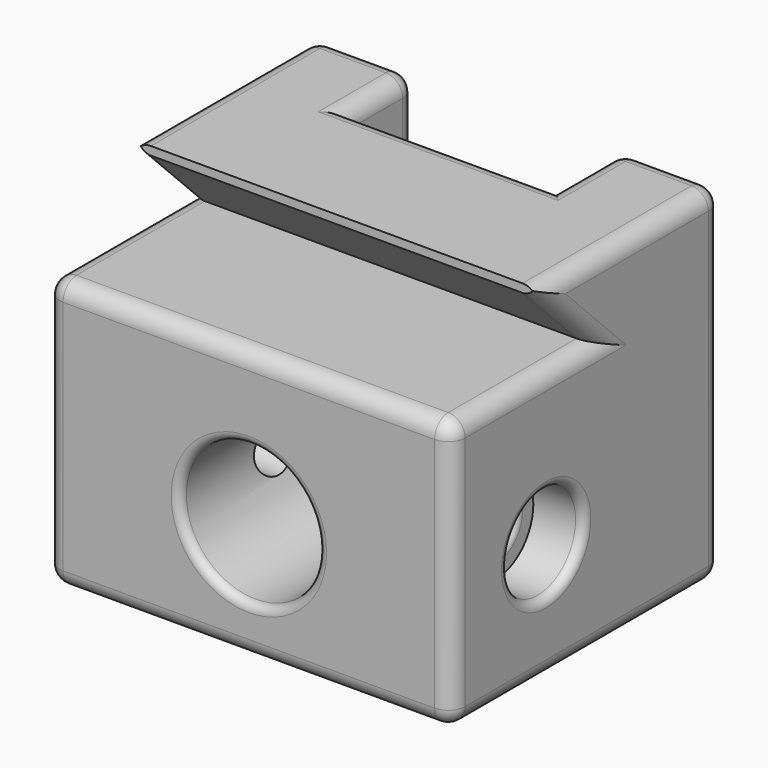
from build123d import *

# Parameters (mm, degrees)
F0_W           = 24
F0_H           = 20
F1_DEPTH       = 18.5
F2_R           = 1.5
F3_DEPTH       = 25
F4_DEPTH       = 2
F5_R           = 4.1
F6_DEPTH       = 25
F7_W           = 12.2
F7_H           = 5
F8_DEPTH       = 25
F9_R           = 2.8
F9_R_2         = 1.5
F10_DEPTH      = 3
F12_DEPTH      = 10.5
F13_T1_DEPTH   = 22
F13_T3_DEPTH   = 15
F13_T5_DEPTH   = 18.5
F13_T7_DEPTH   = 3.9
F13_T9_DEPTH   = 14
F13_T11_DEPTH  = 3.9
F13_T13_DEPTH  = 4
F13_T15_DEPTH  = 12.2
F13_T17_DEPTH  = 18
F13_T19_DEPTH  = 2.75
F13_T21_DEPTH  = 5.5
F13_S25_W      = 1
F13_S25_H      = 1
F13_T26_DEPTH  = 1
F13_S31_W      = 1
F13_S31_H      = 1
F13_T32_DEPTH  = 1
F13_S37_W      = 1
F13_S37_H      = 1
F13_T38_DEPTH  = 1
F13_S43_W      = 1
F13_S43_H      = 1
F13_T44_DEPTH  = 1
F13_S49_W      = 1
F13_S49_H      = 1
F13_T50_DEPTH  = 1
F13_S55_W      = 1
F13_S55_H      = 1
F13_T56_DEPTH  = 1
F13_S61_W      = 1
F13_S61_H      = 1
F13_T62_DEPTH  = 1
F13_S67_W      = 1
F13_S67_H      = 1
F13_T68_DEPTH  = 1
F13_S73_W      = 1
F13_S73_H      = 1
F13_T74_DEPTH  = 1
F13_S79_W      = 1
F13_S79_H      = 1
F13_T80_DEPTH  = 1
F13_S85_W      = 1
F13_S85_H      = 1
F13_T86_DEPTH  = 1
F13_S91_W      = 1
F13_S91_H      = 1
F13_T92_DEPTH  = 1
F13_T98_DEPTH  = 12
F13_T103_DEPTH = 12
F13_T108_DEPTH = 10.6568542495
F13_T113_DEPTH = 10.6568542495
F13_T119_DEPTH = 12
F13_T123_DEPTH = 10.6568542495
F13_T130_DEPTH = 12
F13_T134_DEPTH = 10.6568542495
F13_T141_DEPTH = 6.5
F13_T145_DEPTH = 14.7
F13_T152_DEPTH = 14.7
F13_T156_DEPTH = 6.5
F13_T163_DEPTH = 6.5
F13_T167_DEPTH = 14.7
F13_T174_DEPTH = 6.5
F13_T178_DEPTH = 14.7
F13_T185_DEPTH = 5.25
F13_T189_DEPTH = 8
F13_T196_DEPTH = 8
F13_T200_DEPTH = 5.25
F13_T207_DEPTH = 8
F13_T211_DEPTH = 5.25
F13_T218_DEPTH = 8
F13_T222_DEPTH = 5.25
F14_R          = 0.5


# Not quite as in the source:
# - a fillet or chamfer that OpenCascade refuses, or shapes differently, is made with other operations: its cross-section is extruded or revolved along the edge and cut away or added


with BuildPart() as f1:
    # F0 (on Top) → F1 (new body)
    with BuildSketch(Plane.XY):
        Rectangle(F0_W, F0_H)
    extrude(amount=F1_DEPTH)

    # F2 (on face) → F3 (cut)
    with BuildSketch(Plane(origin=(-12, 0, 0), x_dir=(0, -1, 0), z_dir=(-1, 0, 0))):
        Polygon((-0.5, 14), (10, 14), (10, 18.5), (3.5, 18.5), (3.5, 18), align=None)
        with Locations((3, 5)):
            Circle(F2_R)
    extrude(amount=-F3_DEPTH, mode=Mode.SUBTRACT)

    # F4 (add): a face of the model
    f4_faces = [f1.faces().sort_by_distance(p)[0] for p in [
        (0, 0, 0),
    ]]
    extrude(f4_faces, amount=F4_DEPTH)

    # F5 (on face) → F6 (cut)
    with BuildSketch(Plane.XZ.offset(10)):
        with Locations((0, 5)):
            Circle(F5_R)
    extrude(amount=-F6_DEPTH, mode=Mode.SUBTRACT)

    # F7 (on face) → F8 (cut)
    with BuildSketch(Plane.XY.offset(18.5)):
        with Locations((0, 7.5)):
            Rectangle(F7_W, F7_H)
    extrude(amount=-F8_DEPTH, mode=Mode.SUBTRACT)

    # F9 (on face) → F10 (cut)
    with BuildSketch(Plane.YZ.offset(12)):
        with Locations((-3, 5)):
            Circle(F9_R)
        with Locations((-3, 5)):
            Circle(F9_R_2, mode=Mode.SUBTRACT)
    extrude(amount=-F10_DEPTH, mode=Mode.SUBTRACT)

    # F11 (on face) → F12 (cut)
    with BuildSketch(Plane(origin=(0, 0, -2), x_dir=(1, 0, 0), z_dir=(0, 0, -1))):
        Polygon((-7.05, 0.25), (-7.05, 3), (-7.05, 5.75), (-9.8, 5.75), (-9.8, 0.25), align=None)
    extrude(amount=-F12_DEPTH, mode=Mode.SUBTRACT)

    # F13: fillet of radius 1 on 30 edges, made by hand

    # F13_s2 → F13_t1 (cut)
    with BuildSketch(Plane.YZ.offset(-11)):
        with BuildLine():
            ThreePointArc((-10, 13), (-9.7071067812, 13.7071067812), (-9, 14))
            Line((-9, 14), (-10, 14))
            Line((-10, 14), (-10, 13))
        make_face()
        with BuildLine():
            ThreePointArc((-9, -2), (-9.7071067812, -1.7071067812), (-10, -1))
            Line((-10, -1), (-10, -2))
            Line((-10, -2), (-9, -2))
        make_face()
    extrude(amount=F13_T1_DEPTH, mode=Mode.SUBTRACT)

    # F13_s4 → F13_t3 (cut)
    with BuildSketch(Plane.XZ.offset(-9)):
        with BuildLine():
            ThreePointArc((-11, 18.5), (-11.7071067812, 18.2071067812), (-12, 17.5))
            Line((-12, 17.5), (-12, 18.5))
            Line((-12, 18.5), (-11, 18.5))
        make_face()
        with BuildLine():
            ThreePointArc((12, 17.5), (11.7071067812, 18.2071067812), (11, 18.5))
            Line((11, 18.5), (12, 18.5))
            Line((12, 18.5), (12, 17.5))
        make_face()
    extrude(amount=F13_T3_DEPTH, mode=Mode.SUBTRACT)

    # F13_s6 → F13_t5 (cut)
    with BuildSketch(Plane.XY.offset(-1)):
        with BuildLine():
            ThreePointArc((12, 9), (11.7071067812, 9.7071067812), (11, 10))
            Line((11, 10), (12, 10))
            Line((12, 10), (12, 9))
        make_face()
        with BuildLine():
            ThreePointArc((7.1, 10), (6.3928932188, 9.7071067812), (6.1, 9))
            Line((6.1, 9), (6.1, 10))
            Line((6.1, 10), (7.1, 10))
        make_face()
        with BuildLine():
            ThreePointArc((-7.1, 10), (-6.3928932188, 9.7071067812), (-6.1, 9))
            Line((-6.1, 9), (-6.1, 10))
            Line((-6.1, 10), (-7.1, 10))
        make_face()
        with BuildLine():
            ThreePointArc((-12, 9), (-11.7071067812, 9.7071067812), (-11, 10))
            Line((-11, 10), (-12, 10))
            Line((-12, 10), (-12, 9))
        make_face()
    extrude(amount=F13_T5_DEPTH, mode=Mode.SUBTRACT)

    # F13_s8 → F13_t7 (cut)
    with BuildSketch(Plane.YZ.offset(7.1)):
        with BuildLine():
            ThreePointArc((10, 17.5), (9.7071067812, 18.2071067812), (9, 18.5))
            Line((9, 18.5), (10, 18.5))
            Line((10, 18.5), (10, 17.5))
        make_face()
        with BuildLine():
            ThreePointArc((10, -1), (9.7071067812, -1.7071067812), (9, -2))
            Line((9, -2), (10, -2))
            Line((10, -2), (10, -1))
        make_face()
    extrude(amount=F13_T7_DEPTH, mode=Mode.SUBTRACT)

    # F13_s10 → F13_t9 (cut)
    with BuildSketch(Plane.XY.offset(-1)):
        with BuildLine():
            ThreePointArc((-11, -10), (-11.7071067812, -9.7071067812), (-12, -9))
            Line((-12, -9), (-12, -10))
            Line((-12, -10), (-11, -10))
        make_face()
        with BuildLine():
            ThreePointArc((12, -9), (11.7071067812, -9.7071067812), (11, -10))
            Line((11, -10), (12, -10))
            Line((12, -10), (12, -9))
        make_face()
    extrude(amount=F13_T9_DEPTH, mode=Mode.SUBTRACT)

    # F13_s12 → F13_t11 (cut)
    with BuildSketch(Plane.YZ.offset(-11)):
        with BuildLine():
            ThreePointArc((9, 18.5), (9.7071067812, 18.2071067812), (10, 17.5))
            Line((10, 17.5), (10, 18.5))
            Line((10, 18.5), (9, 18.5))
        make_face()
        with BuildLine():
            ThreePointArc((9, -2), (9.7071067812, -1.7071067812), (10, -1))
            Line((10, -1), (10, -2))
            Line((10, -2), (9, -2))
        make_face()
    extrude(amount=F13_T11_DEPTH, mode=Mode.SUBTRACT)

    # F13_s14 → F13_t13 (cut)
    with BuildSketch(Plane.XZ.offset(-9)):
        with BuildLine():
            ThreePointArc((-7.1, 18.5), (-6.3928932188, 18.2071067812), (-6.1, 17.5))
            Line((-6.1, 17.5), (-6.1, 18.5))
            Line((-6.1, 18.5), (-7.1, 18.5))
        make_face()
        with BuildLine():
            ThreePointArc((7.1, 18.5), (6.3928932188, 18.2071067812), (6.1, 17.5))
            Line((6.1, 17.5), (6.1, 18.5))
            Line((6.1, 18.5), (7.1, 18.5))
        make_face()
        with BuildLine():
            ThreePointArc((-7.1, -2), (-6.3928932188, -1.7071067812), (-6.1, -1))
            Line((-6.1, -1), (-6.1, -2))
            Line((-6.1, -2), (-7.1, -2))
        make_face()
        with BuildLine():
            ThreePointArc((7.1, -2), (6.3928932188, -1.7071067812), (6.1, -1))
            Line((6.1, -1), (6.1, -2))
            Line((6.1, -2), (7.1, -2))
        make_face()
    extrude(amount=F13_T13_DEPTH, mode=Mode.SUBTRACT)

    # F13_s16 → F13_t15 (cut)
    with BuildSketch(Plane.YZ.offset(-6.1)):
        with BuildLine():
            ThreePointArc((4, 18.5), (4.7071067812, 18.2071067812), (5, 17.5))
            Line((5, 17.5), (5, 18.5))
            Line((5, 18.5), (4, 18.5))
        make_face()
        with BuildLine():
            ThreePointArc((4, -2), (4.7071067812, -1.7071067812), (5, -1))
            Line((5, -1), (5, -2))
            Line((5, -2), (4, -2))
        make_face()
    extrude(amount=F13_T15_DEPTH, mode=Mode.SUBTRACT)

    # F13_s18 → F13_t17 (cut)
    with BuildSketch(Plane.XZ.offset(-9)):
        with BuildLine():
            ThreePointArc((12, -1), (11.7071067812, -1.7071067812), (11, -2))
            Line((11, -2), (12, -2))
            Line((12, -2), (12, -1))
        make_face()
        with BuildLine():
            ThreePointArc((-11, -2), (-11.7071067812, -1.7071067812), (-12, -1))
            Line((-12, -1), (-12, -2))
            Line((-12, -2), (-11, -2))
        make_face()
    extrude(amount=F13_T17_DEPTH, mode=Mode.SUBTRACT)

    # F13_s20 → F13_t19 (cut)
    with BuildSketch(Plane.YZ.offset(-9.8)):
        with BuildLine():
            ThreePointArc((0.75, -2), (0.0428932188, -1.7071067812), (-0.25, -1))
            Line((-0.25, -1), (-0.25, -2))
            Line((-0.25, -2), (0.75, -2))
        make_face()
        with BuildLine():
            ThreePointArc((-6.75, -2), (-6.0428932188, -1.7071067812), (-5.75, -1))
            Line((-5.75, -1), (-5.75, -2))
            Line((-5.75, -2), (-6.75, -2))
        make_face()
    extrude(amount=F13_T19_DEPTH, mode=Mode.SUBTRACT)

    # F13_s22 → F13_t21 (cut)
    with BuildSketch(Plane.XZ.offset(0.25)):
        with BuildLine():
            ThreePointArc((-10.8, -2), (-10.0928932188, -1.7071067812), (-9.8, -1))
            Line((-9.8, -1), (-9.8, -2))
            Line((-9.8, -2), (-10.8, -2))
        make_face()
        with BuildLine():
            ThreePointArc((-6.05, -2), (-6.7571067812, -1.7071067812), (-7.05, -1))
            Line((-7.05, -1), (-7.05, -2))
            Line((-7.05, -2), (-6.05, -2))
        make_face()
    extrude(amount=F13_T21_DEPTH, mode=Mode.SUBTRACT)


with BuildPart() as f13_tool24:
    # F13_s25 → F13_t26 (new body)
    with BuildSketch(Plane.YZ.offset(-11)):
        with Locations((-9.5, 13.5)):
            Rectangle(F13_S25_W, F13_S25_H)
    extrude(amount=-F13_T26_DEPTH)

    # F13_s27 → F13_t28 (revolve, cut)
    with BuildSketch(Plane(origin=(-11, -9, 13), x_dir=(0, 0.7071067812, -0.7071067812), z_dir=(0, 0.7071067812, 0.7071067812))):
        with BuildLine():
            ThreePointArc((0, -1), (1, 0), (0, 1))
            Line((0, 1), (0, -1))
        make_face()
    revolve(axis=Axis((-11, -9, 13), (-1, 0, 0)), mode=Mode.SUBTRACT)


with BuildPart() as f1_1:
    add(f1.part)

    # F13_t23: cut F13_tool24
    add(f13_tool24.part, mode=Mode.SUBTRACT)


with BuildPart() as f13_tool30:
    # F13_s31 → F13_t32 (new body)
    with BuildSketch(Plane.YZ.offset(11)):
        with Locations((-9.5, 13.5)):
            Rectangle(F13_S31_W, F13_S31_H)
    extrude(amount=F13_T32_DEPTH)

    # F13_s33 → F13_t34 (revolve, cut)
    with BuildSketch(Plane(origin=(11, -9, 13), x_dir=(0, 0.7071067812, -0.7071067812), z_dir=(0, -0.7071067812, -0.7071067812))):
        with BuildLine():
            ThreePointArc((0, -1), (1, 0), (0, 1))
            Line((0, 1), (0, -1))
        make_face()
    revolve(axis=Axis((11, -9, 13), (1, 0, 0)), mode=Mode.SUBTRACT)


with BuildPart() as f1_2:
    add(f1_1.part)

    # F13_t29: cut F13_tool30
    add(f13_tool30.part, mode=Mode.SUBTRACT)


with BuildPart() as f13_tool36:
    # F13_s37 → F13_t38 (new body)
    with BuildSketch(Plane.XZ.offset(-9)):
        with Locations((-11.5, 18)):
            Rectangle(F13_S37_W, F13_S37_H)
    extrude(amount=-F13_T38_DEPTH)

    # F13_s39 → F13_t40 (revolve, cut)
    with BuildSketch(Plane(origin=(-11, 9, 17.5), x_dir=(0.7071067812, 0, -0.7071067812), z_dir=(0.7071067812, 0, 0.7071067812))):
        with BuildLine():
            ThreePointArc((0, -1), (1, 0), (0, 1))
            Line((0, 1), (0, -1))
        make_face()
    revolve(axis=Axis((-11, 9, 17.5), (0, 1, 0)), mode=Mode.SUBTRACT)


with BuildPart() as f1_3:
    add(f1_2.part)

    # F13_t35: cut F13_tool36
    add(f13_tool36.part, mode=Mode.SUBTRACT)


with BuildPart() as f13_tool42:
    # F13_s43 → F13_t44 (new body)
    with BuildSketch(Plane.YZ.offset(11)):
        with Locations((9.5, 18)):
            Rectangle(F13_S43_W, F13_S43_H)
    extrude(amount=F13_T44_DEPTH)

    # F13_s45 → F13_t46 (revolve, cut)
    with BuildSketch(Plane(origin=(11, 9, 17.5), x_dir=(0, -0.7071067812, -0.7071067812), z_dir=(0, -0.7071067812, 0.7071067812))):
        with BuildLine():
            ThreePointArc((0, -1), (1, 0), (0, 1))
            Line((0, 1), (0, -1))
        make_face()
    revolve(axis=Axis((11, 9, 17.5), (1, 0, 0)), mode=Mode.SUBTRACT)


with BuildPart() as f1_4:
    add(f1_3.part)

    # F13_t41: cut F13_tool42
    add(f13_tool42.part, mode=Mode.SUBTRACT)


with BuildPart() as f13_tool48:
    # F13_s49 → F13_t50 (new body)
    with BuildSketch(Plane.YZ.offset(11)):
        with Locations((9.5, -1.5)):
            Rectangle(F13_S49_W, F13_S49_H)
    extrude(amount=F13_T50_DEPTH)

    # F13_s51 → F13_t52 (revolve, cut)
    with BuildSketch(Plane(origin=(11, 9, -1), x_dir=(0, -0.7071067812, 0.7071067812), z_dir=(0, 0.7071067812, 0.7071067812))):
        with BuildLine():
            ThreePointArc((0, -1), (1, 0), (0, 1))
            Line((0, 1), (0, -1))
        make_face()
    revolve(axis=Axis((11, 9, -1), (1, 0, 0)), mode=Mode.SUBTRACT)


with BuildPart() as f1_5:
    add(f1_4.part)

    # F13_t47: cut F13_tool48
    add(f13_tool48.part, mode=Mode.SUBTRACT)


with BuildPart() as f13_tool54:
    # F13_s55 → F13_t56 (new body)
    with BuildSketch(Plane.XZ.offset(-9)):
        with Locations((6.6, 18)):
            Rectangle(F13_S55_W, F13_S55_H)
    extrude(amount=-F13_T56_DEPTH)

    # F13_s57 → F13_t58 (revolve, cut)
    with BuildSketch(Plane(origin=(7.1, 9, 17.5), x_dir=(0.7071067812, 0, -0.7071067812), z_dir=(0.7071067812, 0, 0.7071067812))):
        with BuildLine():
            ThreePointArc((0, -1), (1, 0), (0, 1))
            Line((0, 1), (0, -1))
        make_face()
    revolve(axis=Axis((7.1, 9, 17.5), (0, 1, 0)), mode=Mode.SUBTRACT)


with BuildPart() as f1_6:
    add(f1_5.part)

    # F13_t53: cut F13_tool54
    add(f13_tool54.part, mode=Mode.SUBTRACT)


with BuildPart() as f13_tool60:
    # F13_s61 → F13_t62 (new body)
    with BuildSketch(Plane.YZ.offset(-11)):
        with Locations((-9.5, -1.5)):
            Rectangle(F13_S61_W, F13_S61_H)
    extrude(amount=-F13_T62_DEPTH)

    # F13_s63 → F13_t64 (revolve, cut)
    with BuildSketch(Plane(origin=(-11, -9, -1), x_dir=(0, 0.7071067812, 0.7071067812), z_dir=(0, -0.7071067812, 0.7071067812))):
        with BuildLine():
            ThreePointArc((0, -1), (1, 0), (0, 1))
            Line((0, 1), (0, -1))
        make_face()
    revolve(axis=Axis((-11, -9, -1), (-1, 0, 0)), mode=Mode.SUBTRACT)


with BuildPart() as f1_7:
    add(f1_6.part)

    # F13_t59: cut F13_tool60
    add(f13_tool60.part, mode=Mode.SUBTRACT)


with BuildPart() as f13_tool66:
    # F13_s67 → F13_t68 (new body)
    with BuildSketch(Plane.YZ.offset(11)):
        with Locations((-9.5, -1.5)):
            Rectangle(F13_S67_W, F13_S67_H)
    extrude(amount=F13_T68_DEPTH)

    # F13_s69 → F13_t70 (revolve, cut)
    with BuildSketch(Plane(origin=(11, -9, -1), x_dir=(0, 0.7071067812, 0.7071067812), z_dir=(0, 0.7071067812, -0.7071067812))):
        with BuildLine():
            ThreePointArc((0, -1), (1, 0), (0, 1))
            Line((0, 1), (0, -1))
        make_face()
    revolve(axis=Axis((11, -9, -1), (1, 0, 0)), mode=Mode.SUBTRACT)


with BuildPart() as f1_8:
    add(f1_7.part)

    # F13_t65: cut F13_tool66
    add(f13_tool66.part, mode=Mode.SUBTRACT)


with BuildPart() as f13_tool72:
    # F13_s73 → F13_t74 (new body)
    with BuildSketch(Plane.XZ.offset(-9)):
        with Locations((-6.6, 18)):
            Rectangle(F13_S73_W, F13_S73_H)
    extrude(amount=-F13_T74_DEPTH)

    # F13_s75 → F13_t76 (revolve, cut)
    with BuildSketch(Plane(origin=(-7.1, 9, 17.5), x_dir=(-0.7071067812, 0, -0.7071067812), z_dir=(0.7071067812, 0, -0.7071067812))):
        with BuildLine():
            ThreePointArc((0, -1), (1, 0), (0, 1))
            Line((0, 1), (0, -1))
        make_face()
    revolve(axis=Axis((-7.1, 9, 17.5), (0, 1, 0)), mode=Mode.SUBTRACT)


with BuildPart() as f1_9:
    add(f1_8.part)

    # F13_t71: cut F13_tool72
    add(f13_tool72.part, mode=Mode.SUBTRACT)


with BuildPart() as f13_tool78:
    # F13_s79 → F13_t80 (new body)
    with BuildSketch(Plane.XZ.offset(-9)):
        with Locations((6.6, -1.5)):
            Rectangle(F13_S79_W, F13_S79_H)
    extrude(amount=-F13_T80_DEPTH)

    # F13_s81 → F13_t82 (revolve, cut)
    with BuildSketch(Plane(origin=(7.1, 9, -1), x_dir=(0.7071067812, 0, 0.7071067812), z_dir=(-0.7071067812, 0, 0.7071067812))):
        with BuildLine():
            ThreePointArc((0, -1), (1, 0), (0, 1))
            Line((0, 1), (0, -1))
        make_face()
    revolve(axis=Axis((7.1, 9, -1), (0, 1, 0)), mode=Mode.SUBTRACT)


with BuildPart() as f1_10:
    add(f1_9.part)

    # F13_t77: cut F13_tool78
    add(f13_tool78.part, mode=Mode.SUBTRACT)


with BuildPart() as f13_tool84:
    # F13_s85 → F13_t86 (new body)
    with BuildSketch(Plane.XY.offset(-1)):
        with Locations((-6.6, 9.5)):
            Rectangle(F13_S85_W, F13_S85_H)
    extrude(amount=-F13_T86_DEPTH)

    # F13_s87 → F13_t88 (revolve, cut)
    with BuildSketch(Plane(origin=(-7.1, 9, -1), x_dir=(-0.7071067812, -0.7071067812, 0), z_dir=(0.7071067812, -0.7071067812, 0))):
        with BuildLine():
            ThreePointArc((0, -1), (1, 0), (0, 1))
            Line((0, 1), (0, -1))
        make_face()
    revolve(axis=Axis((-7.1, 9, -1), (0, 0, -1)), mode=Mode.SUBTRACT)


with BuildPart() as f1_11:
    add(f1_10.part)

    # F13_t83: cut F13_tool84
    add(f13_tool84.part, mode=Mode.SUBTRACT)


with BuildPart() as f13_tool90:
    # F13_s91 → F13_t92 (new body)
    with BuildSketch(Plane.XY.offset(-1)):
        with Locations((-11.5, 9.5)):
            Rectangle(F13_S91_W, F13_S91_H)
    extrude(amount=-F13_T92_DEPTH)

    # F13_s93 → F13_t94 (revolve, cut)
    with BuildSketch(Plane(origin=(-11, 9, -1), x_dir=(0.7071067812, -0.7071067812, 0), z_dir=(0.7071067812, 0.7071067812, 0))):
        with BuildLine():
            ThreePointArc((0, -1), (1, 0), (0, 1))
            Line((0, 1), (0, -1))
        make_face()
    revolve(axis=Axis((-11, 9, -1), (0, 0, -1)), mode=Mode.SUBTRACT)


with BuildPart() as f1_12:
    add(f1_11.part)

    # F13_t89: cut F13_tool90
    add(f13_tool90.part, mode=Mode.SUBTRACT)


with BuildPart() as f13_tool96:
    # F13_s97 → F13_t98 (new body)
    with BuildSketch(Plane.XZ.offset(-3)):
        with BuildLine():
            ThreePointArc((-11, 14), (-11.7071067812, 13.7071067812), (-12, 13))
            Line((-12, 13), (-12, 14))
            Line((-12, 14), (-11, 14))
        make_face()
    extrude(amount=F13_T98_DEPTH)

    split(bisect_by=Plane(origin=(0, 7.25, 7.25), x_dir=(1, 0, 0), z_dir=(0, -0.7071067812, -0.7071067812)), keep=Keep.TOP)


with BuildPart() as f1_13:
    add(f1_12.part)

    # F13_t95: cut F13_tool96
    add(f13_tool96.part, mode=Mode.SUBTRACT)


with BuildPart() as f13_tool101:
    # F13_s102 → F13_t103 (new body)
    with BuildSketch(Plane.XZ.offset(-3)):
        with BuildLine():
            ThreePointArc((12, 13), (11.7071067812, 13.7071067812), (11, 14))
            Line((11, 14), (12, 14))
            Line((12, 14), (12, 13))
        make_face()
    extrude(amount=F13_T103_DEPTH)

    split(bisect_by=Plane(origin=(0, 7.25, 7.25), x_dir=(1, 0, 0), z_dir=(0, -0.7071067812, -0.7071067812)), keep=Keep.TOP)


with BuildPart() as f1_14:
    add(f1_13.part)

    # F13_t100: cut F13_tool101
    add(f13_tool101.part, mode=Mode.SUBTRACT)


with BuildPart() as f13_tool106:
    # F13_s107 → F13_t108 (new body)
    with BuildSketch(Plane(origin=(0, -12.517766953, 12.517766953), x_dir=(1, 0, 0), z_dir=(0, 0.7071067812, -0.7071067812))):
        with BuildLine():
            ThreePointArc((12, -11.2530483272), (11.7071067812, -10.545941546), (11, -10.2530483272))
            Line((11, -10.2530483272), (12, -10.2530483272))
            Line((12, -10.2530483272), (12, -11.2530483272))
        make_face()
    extrude(amount=F13_T108_DEPTH)

    split(bisect_by=Plane.XY.offset(14), keep=Keep.TOP)


with BuildPart() as f1_15:
    add(f1_14.part)

    # F13_t105: cut F13_tool106
    add(f13_tool106.part, mode=Mode.SUBTRACT)


with BuildPart() as f13_tool111:
    # F13_s112 → F13_t113 (new body)
    with BuildSketch(Plane(origin=(0, -12.517766953, 12.517766953), x_dir=(1, 0, 0), z_dir=(0, 0.7071067812, -0.7071067812))):
        with BuildLine():
            ThreePointArc((-11, -10.2530483272), (-11.7071067812, -10.545941546), (-12, -11.2530483272))
            Line((-12, -11.2530483272), (-12, -10.2530483272))
            Line((-12, -10.2530483272), (-11, -10.2530483272))
        make_face()
    extrude(amount=F13_T113_DEPTH)

    split(bisect_by=Plane.XY.offset(14), keep=Keep.TOP)


with BuildPart() as f1_16:
    add(f1_15.part)

    # F13_t110: cut F13_tool111
    add(f13_tool111.part, mode=Mode.SUBTRACT)


with BuildPart() as f13_tool117:
    # F13_s118 → F13_t119 (new body)
    with BuildSketch(Plane.XZ.offset(-3)):
        with BuildLine():
            ThreePointArc((-11, 14), (-11.7071067812, 13.7071067812), (-12, 13))
            Line((-12, 13), (-12, 14))
            Line((-12, 14), (-11, 14))
        make_face()
    extrude(amount=F13_T119_DEPTH)

    split(bisect_by=Plane(origin=(0, 7.25, 7.25), x_dir=(1, 0, 0), z_dir=(0, 0.7071067812, 0.7071067812)), keep=Keep.TOP)


with BuildPart() as f13_tool121:
    # F13_s122 → F13_t123 (new body)
    with BuildSketch(Plane(origin=(0, -12.517766953, 12.517766953), x_dir=(1, 0, 0), z_dir=(0, 0.7071067812, -0.7071067812))):
        with BuildLine():
            ThreePointArc((-11, -10.2530483272), (-11.7071067812, -10.545941546), (-12, -11.2530483272))
            Line((-12, -11.2530483272), (-12, -10.2530483272))
            Line((-12, -10.2530483272), (-11, -10.2530483272))
        make_face()
    extrude(amount=F13_T123_DEPTH)

    split(bisect_by=Plane.XY.offset(14), keep=Keep.BOTTOM)


with BuildPart() as f13_tool117_1:
    add(f13_tool117.part)

    # F13_t125: intersect F13_tool121
    add(f13_tool121.part, mode=Mode.INTERSECT)


with BuildPart() as f1_17:
    add(f1_16.part)

    # F13_t115: cut F13_tool117
    add(f13_tool117_1.part, mode=Mode.SUBTRACT)


with BuildPart() as f13_tool128:
    # F13_s129 → F13_t130 (new body)
    with BuildSketch(Plane.XZ.offset(-3)):
        with BuildLine():
            ThreePointArc((12, 13), (11.7071067812, 13.7071067812), (11, 14))
            Line((11, 14), (12, 14))
            Line((12, 14), (12, 13))
        make_face()
    extrude(amount=F13_T130_DEPTH)

    split(bisect_by=Plane(origin=(0, 7.25, 7.25), x_dir=(1, 0, 0), z_dir=(0, 0.7071067812, 0.7071067812)), keep=Keep.TOP)


with BuildPart() as f13_tool132:
    # F13_s133 → F13_t134 (new body)
    with BuildSketch(Plane(origin=(0, -12.517766953, 12.517766953), x_dir=(1, 0, 0), z_dir=(0, 0.7071067812, -0.7071067812))):
        with BuildLine():
            ThreePointArc((12, -11.2530483272), (11.7071067812, -10.545941546), (11, -10.2530483272))
            Line((11, -10.2530483272), (12, -10.2530483272))
            Line((12, -10.2530483272), (12, -11.2530483272))
        make_face()
    extrude(amount=F13_T134_DEPTH)

    split(bisect_by=Plane.XY.offset(14), keep=Keep.BOTTOM)


with BuildPart() as f13_tool128_1:
    add(f13_tool128.part)

    # F13_t136: intersect F13_tool132
    add(f13_tool132.part, mode=Mode.INTERSECT)


with BuildPart() as f1_18:
    add(f1_17.part)

    # F13_t126: cut F13_tool128
    add(f13_tool128_1.part, mode=Mode.SUBTRACT)


with BuildPart() as f13_tool139:
    # F13_s140 → F13_t141 (new body)
    with BuildSketch(Plane.XZ.offset(-9)):
        with BuildLine():
            ThreePointArc((-7.1, 18.5), (-6.3928932188, 18.2071067812), (-6.1, 17.5))
            Line((-6.1, 17.5), (-6.1, 18.5))
            Line((-6.1, 18.5), (-7.1, 18.5))
        make_face()
    extrude(amount=F13_T141_DEPTH)

    split(bisect_by=Plane.XZ.offset(-5), keep=Keep.TOP)


with BuildPart() as f13_tool143:
    # F13_s144 → F13_t145 (new body)
    with BuildSketch(Plane.YZ.offset(-8.6)):
        with BuildLine():
            ThreePointArc((4, 18.5), (4.7071067812, 18.2071067812), (5, 17.5))
            Line((5, 17.5), (5, 18.5))
            Line((5, 18.5), (4, 18.5))
        make_face()
    extrude(amount=F13_T145_DEPTH)

    split(bisect_by=Plane.YZ.offset(-6.1), keep=Keep.BOTTOM)


with BuildPart() as f13_tool139_1:
    add(f13_tool139.part)

    # F13_t147: intersect F13_tool143
    add(f13_tool143.part, mode=Mode.INTERSECT)


with BuildPart() as f1_19:
    add(f1_18.part)

    # F13_t137: cut F13_tool139
    add(f13_tool139_1.part, mode=Mode.SUBTRACT)


with BuildPart() as f13_tool150:
    # F13_s151 → F13_t152 (new body)
    with BuildSketch(Plane.YZ.offset(-6.1)):
        with BuildLine():
            ThreePointArc((4, 18.5), (4.7071067812, 18.2071067812), (5, 17.5))
            Line((5, 17.5), (5, 18.5))
            Line((5, 18.5), (4, 18.5))
        make_face()
    extrude(amount=F13_T152_DEPTH)

    split(bisect_by=Plane.YZ.offset(6.1), keep=Keep.TOP)


with BuildPart() as f13_tool154:
    # F13_s155 → F13_t156 (new body)
    with BuildSketch(Plane.XZ.offset(-2.5)):
        with BuildLine():
            ThreePointArc((7.1, 18.5), (6.3928932188, 18.2071067812), (6.1, 17.5))
            Line((6.1, 17.5), (6.1, 18.5))
            Line((6.1, 18.5), (7.1, 18.5))
        make_face()
    extrude(amount=-F13_T156_DEPTH)

    split(bisect_by=Plane.XZ.offset(-5), keep=Keep.TOP)


with BuildPart() as f13_tool150_1:
    add(f13_tool150.part)

    # F13_t158: intersect F13_tool154
    add(f13_tool154.part, mode=Mode.INTERSECT)


with BuildPart() as f1_20:
    add(f1_19.part)

    # F13_t148: cut F13_tool150
    add(f13_tool150_1.part, mode=Mode.SUBTRACT)


with BuildPart() as f13_tool161:
    # F13_s162 → F13_t163 (new body)
    with BuildSketch(Plane.XZ.offset(-9)):
        with BuildLine():
            ThreePointArc((-7.1, -2), (-6.3928932188, -1.7071067812), (-6.1, -1))
            Line((-6.1, -1), (-6.1, -2))
            Line((-6.1, -2), (-7.1, -2))
        make_face()
    extrude(amount=F13_T163_DEPTH)

    split(bisect_by=Plane.XZ.offset(-5), keep=Keep.TOP)


with BuildPart() as f13_tool165:
    # F13_s166 → F13_t167 (new body)
    with BuildSketch(Plane.YZ.offset(-8.6)):
        with BuildLine():
            ThreePointArc((4, -2), (4.7071067812, -1.7071067812), (5, -1))
            Line((5, -1), (5, -2))
            Line((5, -2), (4, -2))
        make_face()
    extrude(amount=F13_T167_DEPTH)

    split(bisect_by=Plane.YZ.offset(-6.1), keep=Keep.BOTTOM)


with BuildPart() as f13_tool161_1:
    add(f13_tool161.part)

    # F13_t169: intersect F13_tool165
    add(f13_tool165.part, mode=Mode.INTERSECT)


with BuildPart() as f1_21:
    add(f1_20.part)

    # F13_t159: cut F13_tool161
    add(f13_tool161_1.part, mode=Mode.SUBTRACT)


with BuildPart() as f13_tool172:
    # F13_s173 → F13_t174 (new body)
    with BuildSketch(Plane.XZ.offset(-2.5)):
        with BuildLine():
            ThreePointArc((7.1, -2), (6.3928932188, -1.7071067812), (6.1, -1))
            Line((6.1, -1), (6.1, -2))
            Line((6.1, -2), (7.1, -2))
        make_face()
    extrude(amount=-F13_T174_DEPTH)

    split(bisect_by=Plane.XZ.offset(-5), keep=Keep.TOP)


with BuildPart() as f13_tool176:
    # F13_s177 → F13_t178 (new body)
    with BuildSketch(Plane.YZ.offset(-6.1)):
        with BuildLine():
            ThreePointArc((4, -2), (4.7071067812, -1.7071067812), (5, -1))
            Line((5, -1), (5, -2))
            Line((5, -2), (4, -2))
        make_face()
    extrude(amount=F13_T178_DEPTH)

    split(bisect_by=Plane.YZ.offset(6.1), keep=Keep.TOP)


with BuildPart() as f13_tool172_1:
    add(f13_tool172.part)

    # F13_t180: intersect F13_tool176
    add(f13_tool176.part, mode=Mode.INTERSECT)


with BuildPart() as f1_22:
    add(f1_21.part)

    # F13_t170: cut F13_tool172
    add(f13_tool172_1.part, mode=Mode.SUBTRACT)


with BuildPart() as f13_tool183:
    # F13_s184 → F13_t185 (new body)
    with BuildSketch(Plane.YZ.offset(-12.3)):
        with BuildLine():
            ThreePointArc((0.75, -2), (0.0428932188, -1.7071067812), (-0.25, -1))
            Line((-0.25, -1), (-0.25, -2))
            Line((-0.25, -2), (0.75, -2))
        make_face()
    extrude(amount=F13_T185_DEPTH)

    split(bisect_by=Plane.YZ.offset(-9.8), keep=Keep.BOTTOM)


with BuildPart() as f13_tool187:
    # F13_s188 → F13_t189 (new body)
    with BuildSketch(Plane.XZ.offset(5.75)):
        with BuildLine():
            ThreePointArc((-10.8, -2), (-10.0928932188, -1.7071067812), (-9.8, -1))
            Line((-9.8, -1), (-9.8, -2))
            Line((-9.8, -2), (-10.8, -2))
        make_face()
    extrude(amount=-F13_T189_DEPTH)

    split(bisect_by=Plane.XZ.offset(0.25), keep=Keep.BOTTOM)


with BuildPart() as f13_tool183_1:
    add(f13_tool183.part)

    # F13_t191: intersect F13_tool187
    add(f13_tool187.part, mode=Mode.INTERSECT)


with BuildPart() as f1_23:
    add(f1_22.part)

    # F13_t181: cut F13_tool183
    add(f13_tool183_1.part, mode=Mode.SUBTRACT)


with BuildPart() as f13_tool194:
    # F13_s195 → F13_t196 (new body)
    with BuildSketch(Plane.XZ.offset(5.75)):
        with BuildLine():
            ThreePointArc((-6.05, -2), (-6.7571067812, -1.7071067812), (-7.05, -1))
            Line((-7.05, -1), (-7.05, -2))
            Line((-7.05, -2), (-6.05, -2))
        make_face()
    extrude(amount=-F13_T196_DEPTH)

    split(bisect_by=Plane.XZ.offset(0.25), keep=Keep.BOTTOM)


with BuildPart() as f13_tool198:
    # F13_s199 → F13_t200 (new body)
    with BuildSketch(Plane.YZ.offset(-9.8)):
        with BuildLine():
            ThreePointArc((0.75, -2), (0.0428932188, -1.7071067812), (-0.25, -1))
            Line((-0.25, -1), (-0.25, -2))
            Line((-0.25, -2), (0.75, -2))
        make_face()
    extrude(amount=F13_T200_DEPTH)

    split(bisect_by=Plane.YZ.offset(-7.05), keep=Keep.TOP)


with BuildPart() as f13_tool194_1:
    add(f13_tool194.part)

    # F13_t202: intersect F13_tool198
    add(f13_tool198.part, mode=Mode.INTERSECT)


with BuildPart() as f1_24:
    add(f1_23.part)

    # F13_t192: cut F13_tool194
    add(f13_tool194_1.part, mode=Mode.SUBTRACT)


with BuildPart() as f13_tool205:
    # F13_s206 → F13_t207 (new body)
    with BuildSketch(Plane.XZ.offset(8.25)):
        with BuildLine():
            ThreePointArc((-10.8, -2), (-10.0928932188, -1.7071067812), (-9.8, -1))
            Line((-9.8, -1), (-9.8, -2))
            Line((-9.8, -2), (-10.8, -2))
        make_face()
    extrude(amount=-F13_T207_DEPTH)

    split(bisect_by=Plane.XZ.offset(5.75), keep=Keep.TOP)


with BuildPart() as f13_tool209:
    # F13_s210 → F13_t211 (new body)
    with BuildSketch(Plane.YZ.offset(-7.05)):
        with BuildLine():
            ThreePointArc((-6.75, -2), (-6.0428932188, -1.7071067812), (-5.75, -1))
            Line((-5.75, -1), (-5.75, -2))
            Line((-5.75, -2), (-6.75, -2))
        make_face()
    extrude(amount=-F13_T211_DEPTH)

    split(bisect_by=Plane.YZ.offset(-9.8), keep=Keep.BOTTOM)


with BuildPart() as f13_tool205_1:
    add(f13_tool205.part)

    # F13_t213: intersect F13_tool209
    add(f13_tool209.part, mode=Mode.INTERSECT)


with BuildPart() as f1_25:
    add(f1_24.part)

    # F13_t203: cut F13_tool205
    add(f13_tool205_1.part, mode=Mode.SUBTRACT)


with BuildPart() as f13_tool216:
    # F13_s217 → F13_t218 (new body)
    with BuildSketch(Plane.XZ.offset(8.25)):
        with BuildLine():
            ThreePointArc((-6.05, -2), (-6.7571067812, -1.7071067812), (-7.05, -1))
            Line((-7.05, -1), (-7.05, -2))
            Line((-7.05, -2), (-6.05, -2))
        make_face()
    extrude(amount=-F13_T218_DEPTH)

    split(bisect_by=Plane.XZ.offset(5.75), keep=Keep.TOP)


with BuildPart() as f13_tool220:
    # F13_s221 → F13_t222 (new body)
    with BuildSketch(Plane.YZ.offset(-4.55)):
        with BuildLine():
            ThreePointArc((-6.75, -2), (-6.0428932188, -1.7071067812), (-5.75, -1))
            Line((-5.75, -1), (-5.75, -2))
            Line((-5.75, -2), (-6.75, -2))
        make_face()
    extrude(amount=-F13_T222_DEPTH)

    split(bisect_by=Plane.YZ.offset(-7.05), keep=Keep.TOP)


with BuildPart() as f13_tool216_1:
    add(f13_tool216.part)

    # F13_t224: intersect F13_tool220
    add(f13_tool220.part, mode=Mode.INTERSECT)


with BuildPart() as f1_26:
    add(f1_25.part)

    # F13_t214: cut F13_tool216
    add(f13_tool216_1.part, mode=Mode.SUBTRACT)

    # F14
    f14_edges = [f1_26.edges().sort_by_distance(p)[0] for p in [
        (12, -5.8, 5),
        (-4.1, -10, 5),
        (-4.1, 5, 5),
        (-12, -1.5, 5),
        (11, 0, -2),
        (9, -1.5, 5),
    ]]
    fillet(f14_edges, radius=F14_R)


solid = f1_26.part
